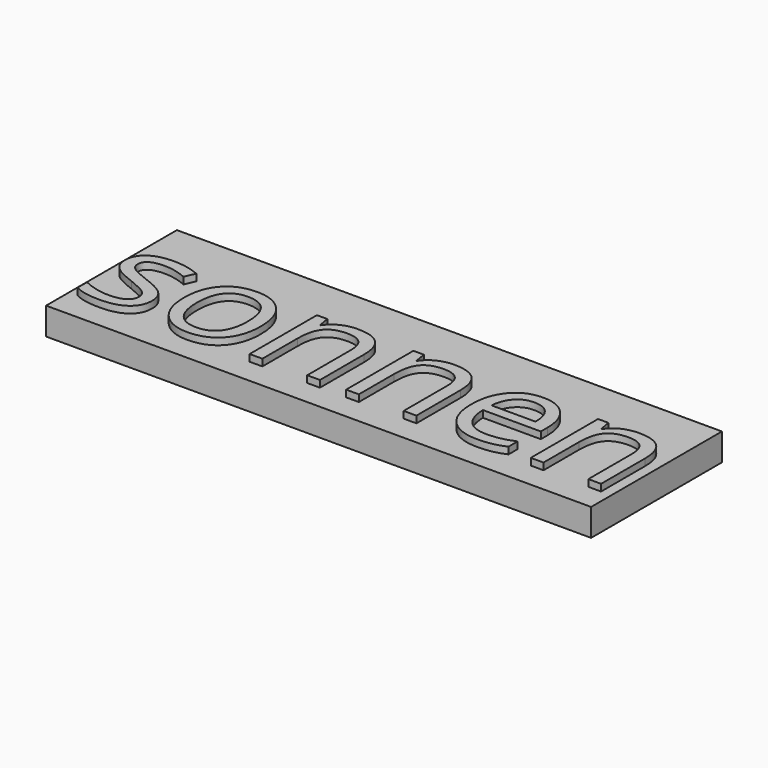
from build123d import *

# Parameters (mm, degrees)
F0_W         = 127
F0_H         = 38.1
F1_DEPTH     = 6.35
F2_TEXT_SIZE = 36.6225105884
F3_DEPTH     = 1.5875


# Not quite as in the source:
# - Text() gives the source's letters only with a copy of the font that has no kerning and outlines rounded to 1/6400 em; it was checked with that copy


with BuildPart() as f1:
    # F0 (on Top) → F1 (new body)
    with BuildSketch(Plane.XY):
        Rectangle(F0_W, F0_H)
    extrude(amount=F1_DEPTH)

    # F2 (on face) → F3 (join)
    with BuildSketch(Plane.XY.offset(6.35)):
        with Locations((-63.5, -13.1841038118)):
            Text('sonnen', F2_TEXT_SIZE, font='Open Sans', text_align=(TextAlign.LEFT, TextAlign.BOTTOM))
    extrude(amount=F3_DEPTH)


solid = f1.part
